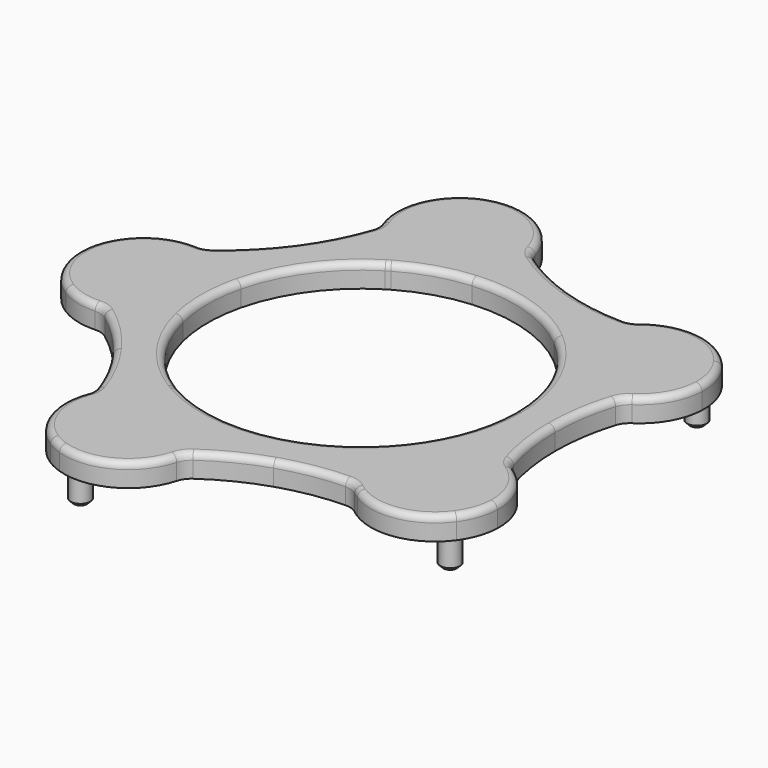
from build123d import *

# Parameters (mm, degrees)
F0_R     = 1.5
F1_DEPTH = 3.5
F2_DEPTH = 5
F3_SIZE  = 0.5
F4_R     = 3
F5_R     = 1


# Not quite as in the source:
# - ends of sketch curves that miss each other by under 0.0002 mm in the source are joined


with BuildPart() as f1:
    # F0 (on Top) → F1 (new body)
    with BuildSketch(Plane.XY):
        with BuildLine():
            ThreePointArc((20.1217779995, 26.6680890251), (14.590298866, 27.0280584449), (9.194486034, 28.2977211047))
            ThreePointArc((9.194486034, 28.2977211047), (4.0828932755, 30.44212139), (-0.6037516551, 33.4022214571))
            ThreePointArc((-0.6037516551, 33.4022214571), (-5.2120993734, 40.198926756), (-13.3690430913, 41.1456836959))
            ThreePointArc((-13.3690430913, 41.1456836959), (-14.1649443957, 40.8485796085), (-14.9323019348, 40.4840358767))
            ThreePointArc((-14.9323019348, 40.4840358767), (-19.7062395311, 34.7883712808), (-19.1448881243, 27.3778409381))
            ThreePointArc((-19.1448881243, 27.3778409381), (-21.1965599583, 22.2283283649), (-24.0714787844, 17.4889528433))
            ThreePointArc((-24.0714787844, 17.4889528433), (-27.6904938656, 13.2901952695), (-31.9539694749, 9.747652249))
            ThreePointArc((-31.9539694749, 9.747652249), (-35.0681057259, 9.714575117), (-38.0164389348, 8.7114468767))
            ThreePointArc((-38.0164389348, 8.7114468767), (-41.8501718559, 5.0847098112), (-43.263132, 3.74e-08))
            ThreePointArc((-43.263132, 3.74e-08), (-42.0324124779, -4.7690597809), (-38.6476309704, -8.3470279528))
            ThreePointArc((-38.6476309704, -8.3470279528), (-35.4261798274, -9.6465351082), (-31.9539699274, -9.7476524868))
            ThreePointArc((-31.9539699274, -9.7476524868), (-27.690493577, -13.2901945529), (-24.0714783088, -17.4889524978))
            ThreePointArc((-24.0714783088, -17.4889524978), (-21.1965597779, -22.228327727), (-19.1448875967, -27.377839877))
            ThreePointArc((-19.1448875967, -27.377839877), (-19.8113357478, -34.4393697881), (-15.5634939704, -40.1196159528))
            ThreePointArc((-15.5634939704, -40.1196159528), (-14.4979147358, -40.7003306499), (-13.3690434722, -41.1456825721))
            ThreePointArc((-13.3690434722, -41.1456825721), (-5.2120999662, -40.1989261156), (-0.6037514608, -33.4022210904))
            ThreePointArc((-0.6037514608, -33.4022210904), (4.0828930084, -30.4421205291), (9.194486034, -28.2977201047))
            ThreePointArc((9.194486034, -28.2977201047), (14.590298866, -27.0280574449), (20.1217779995, -26.6680880251))
            ThreePointArc((20.1217779995, -26.6680880251), (20.9190851421, -27.3707973109), (21.7874240296, -27.9835669528))
            ThreePointArc((21.7874240296, -27.9835669528), (28.8978336404, -29.3128703789), (35.0006086726, -25.4294299793))
            ThreePointArc((35.0006086726, -25.4294299793), (36.3425546535, -22.8548424618), (36.8760932483, -20.0009580092))
            ThreePointArc((36.8760932483, -20.0009580092), (35.5467924692, -14.6817866996), (31.5808301778, -10.8960546587))
            ThreePointArc((31.5808301778, -10.8960546587), (30.2138608068, -5.5240696015), (29.753984, 0))
            ThreePointArc((29.753984, 0), (30.2138608849, 5.5240700677), (31.5808305726, 10.8960558025))
            ThreePointArc((31.5808305726, 10.8960558025), (35.3577575985, 14.3701589843), (36.8760932483, 19.2721209908))
            ThreePointArc((36.8760932483, 19.2721209908), (36.4551855196, 22.5082013015), (35.000608448, 25.4294312884))
            ThreePointArc((35.000608448, 25.4294312884), (29.2543503151, 29.2370914198), (22.4186168465, 28.3479872901))
            ThreePointArc((22.4186168465, 28.3479872901), (21.2092474707, 27.5913718902), (20.1217779995, 26.6680890251))
        make_face()
        with Locations((-12.441992, -38.292513)):
            Circle(F0_R, mode=Mode.SUBTRACT)
        with Locations((32.573558, -23.666075)):
            Circle(F0_R, mode=Mode.SUBTRACT)
        with Locations((-40.263132, 0)):
            Circle(F0_R, mode=Mode.SUBTRACT)
        with Locations((-12.441992, 38.292514)):
            Circle(F0_R, mode=Mode.SUBTRACT)
        with BuildLine():
            ThreePointArc((23.552222, 0), (23.105799083, -4.563902921), (21.7834538666, -8.9547919451))
            ThreePointArc((21.7834538666, -8.9547919451), (19.0541480894, -13.8436484254), (15.2479712846, -17.950112335))
            ThreePointArc((15.2479712846, -17.950112335), (7.2780371129, -22.399494122), (-1.7850560471, -23.4844786198))
            ThreePointArc((-1.7850560471, -23.4844786198), (-6.9541153125, -22.5021652593), (-11.7761112458, -20.3968224257))
            ThreePointArc((-11.7761112458, -20.3968224257), (-12.0691566841, -20.2248020528), (-12.3596898329, -20.048571729))
            ThreePointArc((-12.3596898329, -20.048571729), (-19.0541479048, -13.8436486794), (-22.8866790302, -5.5594140073))
            ThreePointArc((-22.8866790302, -5.5594140073), (-23.552222, 0), (-22.8866790302, 5.5594140073))
            ThreePointArc((-22.8866790302, 5.5594140073), (-19.0541479048, 13.8436486794), (-12.3596898329, 20.048571729))
            ThreePointArc((-12.3596898329, 20.048571729), (-12.0691564694, 20.2248021809), (-11.7761108128, 20.3968226757))
            ThreePointArc((-11.7761108128, 20.3968226757), (-6.9541150375, 22.5021653443), (-1.7850559715, 23.4844786256))
            ThreePointArc((-1.7850559715, 23.4844786256), (7.2780368411, 22.3994942103), (15.2479707912, 17.9501127542))
            ThreePointArc((15.2479707912, 17.9501127542), (19.0541476273, 13.8436490614), (21.7834535149, 8.9547928006))
            ThreePointArc((21.7834535149, 8.9547928006), (23.1057989934, 4.5639033747), (23.552222, 0))
        make_face(mode=Mode.SUBTRACT)
        with Locations((32.573558, 23.666076)):
            Circle(F0_R, mode=Mode.SUBTRACT)
        with Locations((32.573558, 23.666076)):
            Circle(F0_R)
        with Locations((-12.441992, 38.292514)):
            Circle(F0_R)
        with Locations((-40.263132, 0)):
            Circle(F0_R)
        with Locations((-12.441992, -38.292513)):
            Circle(F0_R)
        with Locations((32.573558, -23.666075)):
            Circle(F0_R)
    extrude(amount=F1_DEPTH)

    # F0 (on Top) → F2 (join)
    with BuildSketch(Plane.XY):
        with Locations((-12.441992, 38.292514)):
            Circle(F0_R)
        with Locations((-40.263132, 0)):
            Circle(F0_R)
        with Locations((32.573558, 23.666076)):
            Circle(F0_R)
        with Locations((32.573558, -23.666075)):
            Circle(F0_R)
        with Locations((-12.441992, -38.292513)):
            Circle(F0_R)
    extrude(amount=-F2_DEPTH)

    # F3
    f3_edges = [f1.edges().sort_by_distance(p)[0] for p in [
        (31.073558, -23.666075, -5),
        (31.073558, 23.666076, -5),
        (-13.941992, 38.292514, -5),
        (-41.763132, 0, -5),
        (-13.941992, -38.292513, -5),
    ]]
    chamfer(f3_edges, length=F3_SIZE)

    # F4
    f4_edges = [f1.edges().sort_by_distance(p)[0] for p in [
        (-31.95397, -9.747652, 1.75),
        (-0.603751, -33.402221, 1.75),
        (20.121778, -26.668088, 1.75),
        (-19.144888, -27.37784, 1.75),
        (-31.953969, 9.747652, 1.75),
        (-19.144888, 27.377841, 1.75),
        (-0.603752, 33.402221, 1.75),
        (20.121778, 26.668089, 1.75),
        (31.580831, 10.896056, 1.75),
        (31.58083, -10.896055, 1.75),
    ]]
    fillet(f4_edges, radius=F4_R)

    # F5
    f5_edges = [f1.edges().sort_by_distance(p)[0] for p in [
        (21.616825, 27.87401, 3.5),
        (19.956655, 26.828286, 3.5),
        (32.267332, 27.983568, 3.5),
        (9.194487, 28.297721, 3.5),
        (35.612161, 14.795932, 3.5),
        (-0.376003, 33.434766, 3.5),
        (31.682161, 10.689511, 3.5),
        (-5.642504, 40.445414, 3.5),
        (30.120913, 4.937801, 3.5),
        (-19.208337, 36.037608, 3.5),
        (30.120913, -4.937801, 3.5),
        (-19.34827, 27.270303, 3.5),
        (31.682161, -10.689509, 3.5),
        (-21.465964, 21.699394, 3.5),
        (35.320645, -24.961172, 3.5),
        (-27.270698, 13.709864, 3.5),
        (21.315933, -27.668313, 3.5),
        (-31.914543, 9.974311, 3.5),
        (19.956655, -26.828285, 3.5),
        (-35.554746, 9.618736, 3.5),
        (14.004002, -27.120826, 3.5),
        (-42.913929, -2.600224, 3.5),
        (4.611745, -30.172555, 3.5),
        (-31.914544, -9.974311, 3.5),
        (-0.376003, -33.434766, 3.5),
        (-27.270697, -13.709863, 3.5),
        (-6.743887, -40.954967, 3.5),
        (-21.465964, -21.699393, 3.5),
        (-19.665154, -34.913326, 3.5),
        (-19.34827, -27.270302, 3.5),
        (-21.783454, 8.954792, 3.5),
    ]]
    fillet(f5_edges, radius=F5_R)


solid = f1.part
